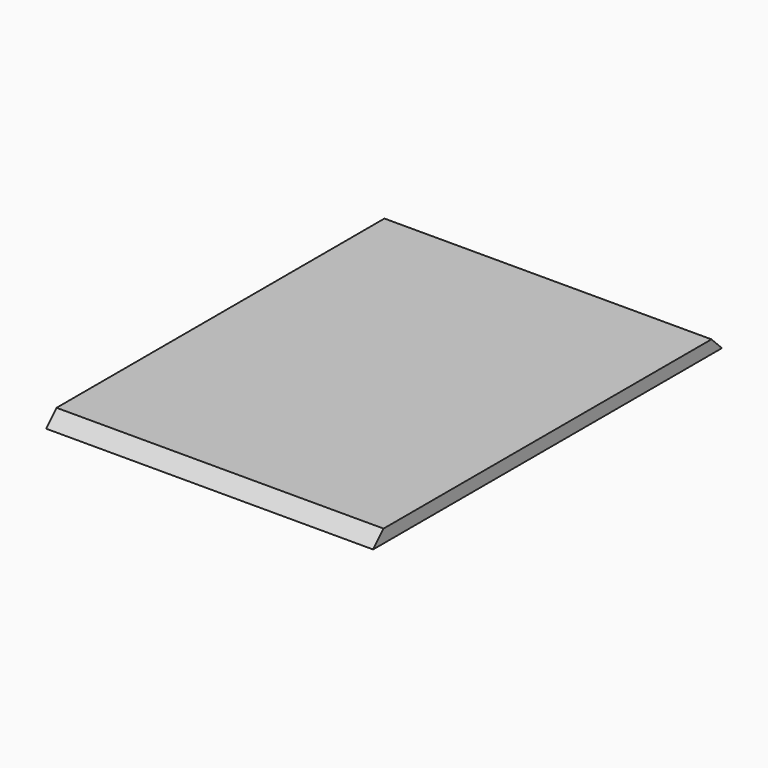
from build123d import *

# Parameters (mm, degrees)
F0_W     = 150
F0_H     = 200
F1_DEPTH = 6
F2_SIZE  = 5.99999


# Not quite as in the source:
# - a fillet or chamfer is up to 0.001 mm smaller than in the source, because OpenCascade refuses the exact size


with BuildPart() as f1:
    # F0 (on Top) → F1 (new body)
    with BuildSketch(Plane.XY):
        with Locations((3.189206589, -5.372708199)):
            Rectangle(F0_W, F0_H)
    extrude(amount=F1_DEPTH)

    # F2 (size 6 in the source; OpenCascade refuses exactly that, so slightly less here)
    f2_edges = [f1.edges().sort_by_distance(p)[0] for p in [
        (3.189207, -105.372708, 6),
        (3.189207, 94.627292, 6),
    ]]
    chamfer(f2_edges, length=F2_SIZE)


solid = f1.part
